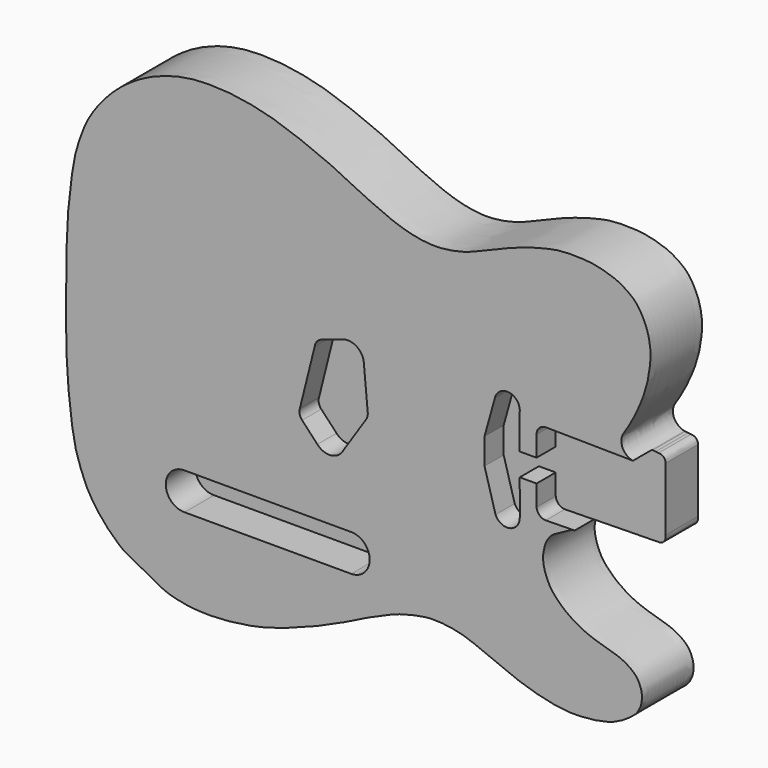
from build123d import *

# Parameters (mm, degrees)
F1_DEPTH = 44.45
F2_DEPTH = 16.51
F3_DEPTH = 25.4


# Not quite as in the source:
# - a feature names something its author has since deleted; it is built from what else it names


with BuildPart() as f1:
    # F0 (on Front) → F1 (new body)
    with BuildSketch(Plane.XZ):
        with BuildLine():
            Line((-36.4628359675, 9.569167666), (-36.4628359675, 27.653967666))
            Line((-36.4628359675, 27.653967666), (-29.3169317005, 53.3077017051))
            ThreePointArc((-29.3169317005, 53.3077017051), (-20.290639837, 59.8672852359), (-12.2146032714, 52.1679531679))
            ThreePointArc((-12.2146032714, 52.1679531679), (-12.1577623785, 51.1793421532), (-12.2134742813, 50.190666873))
            Line((-12.2134742813, 50.190666873), (-12.1998377178, 26.3079138094))
            Line((-12.1998377178, 26.3079138094), (-0.6035441244, 26.3145350559))
            Line((-0.6035441244, 26.3145350559), (-0.6116200717, 40.4585571406))
            ThreePointArc((-0.6116200717, 40.4585571406), (1.2332374634, 44.9781868251), (5.7391212323, 46.856367666))
            Line((5.7391212323, 46.856367666), (65.8569202223, 46.101456937))
            add(Edge.make_bspline(
                [(65.8569202223, 46.101456937), (65.8082198952, 46.111538896), (64.440532792, 46.4005697996), (61.9493146455, 47.2777107227), (58.8086310676, 50.8096057402), (58.0449342483, 53.2991789854), (57.7457666161, 55.8465865019), (58.1162605807, 57.8853867085), (58.8767369784, 60.1253918133), (61.8338810554, 64.2452496747), (64.7748667663, 69.5266396192), (66.9437975867, 73.5325947729), (72.1748619169, 84.4879171866), (75.4157897662, 95.0217528485), (77.0913434636, 102.553719941), (78.8679716791, 117.435063011), (75.0176091289, 132.0874660401), (69.4399127098, 141.1287497127), (66.1646213257, 144.6638685914), (63.8949883169, 146.3744088303), (62.1099414236, 147.7625127314), (59.4477178127, 149.4698385607), (54.8171025343, 152.3289323071), (42.9175321679, 156.1236739531), (32.4036601977, 157.5651964451), (17.2088000215, 157.6253069579), (8.7386710867, 156.0609973015), (-0.497068574, 153.8336518936), (-9.0925484925, 151.2124734508), (-14.4383316219, 149.3290323967), (-22.7118669356, 146.2487000901), (-30.085330014, 142.9097204574), (-39.2612302691, 139.405533864), (-44.8381827502, 136.8638580798), (-51.0647950461, 134.7130453138), (-57.3869608629, 133.2537734899), (-64.5951798295, 132.1353574656), (-72.0653943408, 131.7504818884), (-80.9431789181, 132.7258780715), (-89.4749993511, 134.5505711219), (-99.5171332769, 137.7395440421), (-110.0450246922, 142.4219643584), (-120.9610931472, 147.1972742288), (-134.7691497671, 154.4003080602), (-143.6538012671, 158.4762100092), (-157.5356445432, 164.4053701436), (-175.0197441359, 170.8243226408), (-186.3921154716, 174.3329000019), (-200.859238688, 177.4783450729), (-215.2049744258, 179.3443999642), (-230.3357113691, 179.662308746), (-239.3667204013, 178.8311843075), (-249.7475334686, 176.9580035132), (-258.4388184787, 174.3472655237), (-270.2077546423, 169.617132441), (-281.0330383343, 162.8807350814), (-288.724798983, 156.9716403119), (-296.6119448079, 149.4701577517), (-303.1036787906, 141.6394488957), (-307.9726093768, 134.3784922093), (-311.0811868302, 128.8371006588), (-314.2426482545, 121.1107032616), (-316.6817846786, 114.2377347901), (-319.5777590699, 103.8792354228), (-321.3560431534, 90.7754208806), (-323.3080358572, 75.4582008588), (-324.489070044, 56.0206486034), (-324.9329261688, 30.5273308203), (-325.5213201034, -24.6300824924), (-319.9524725281, -65.9891758085), (-317.0048781693, -76.3928819812), (-311.8939305277, -90.882381175), (-307.2717097261, -98.41395875), (-303.607968046, -103.8373952444), (-299.7301097702, -108.687657352), (-296.0407497518, -113.0005548798), (-290.6753655124, -118.1196416132), (-287.5886005429, -120.701802204), (-285.8139366616, -122.1753017859), (-282.0775126279, -124.3005591876), (-282.0559417692, -124.3111405134)],
                knots=[0.0087884076, 0.0087884076, 0.0087884076, 0.0087884076, 0.0090969709, 0.0174847617, 0.0264572155, 0.033290393, 0.0399451027, 0.0459262298, 0.0522794931, 0.0618231279, 0.0721557838, 0.0812308835, 0.0958978339, 0.1100252966, 0.1217227111, 0.137900103, 0.1545955669, 0.1682230193, 0.1772998584, 0.1842364833, 0.190505402, 0.1977901906, 0.2076124061, 0.2223668275, 0.236629285, 0.2528933764, 0.2654267623, 0.2784218192, 0.2910050259, 0.3011351249, 0.3134791399, 0.3258152578, 0.3389588282, 0.3495071237, 0.360198775, 0.3710109583, 0.382368356, 0.3939634128, 0.4065222933, 0.4190404883, 0.4327282508, 0.4470084074, 0.4618293926, 0.4783570386, 0.49162608, 0.5080146132, 0.5263183465, 0.541010961, 0.5570360296, 0.573418106, 0.5897148303, 0.6025488734, 0.6160172189, 0.6288300734, 0.6438764778, 0.6590024815, 0.672177919, 0.6860518531, 0.6996679541, 0.7120327874, 0.7227283038, 0.7347664787, 0.746248908, 0.759964096, 0.7753743112, 0.79200234, 0.8102768483, 0.8316179392, 0.863706102, 0.8907241456, 0.9045658341, 0.9207868975, 0.9334891204, 0.9441601708, 0.9545570424, 0.9647955615, 0.976344898, 0.984586996, 0.9917273903, 1, 1, 1, 1], degree=3))
            Line((-282.0559417692, -124.3111405134), (-258.0415796527, -137.131692276))
            add(Edge.make_bspline(
                [(-258.0415796527, -137.131692276), (-256.9812734982, -137.60730777), (-254.5368163321, -138.7038040014), (-248.166441932, -140.3729487716), (-242.3794546895, -141.4900264019), (-236.1497706051, -142.2474812095), (-230.1384817638, -142.644410985), (-222.0753688735, -142.5836604529), (-213.2788451825, -142.0513216814), (-204.1233965754, -140.9044073657), (-193.5549385183, -139.0785143182), (-184.0685444079, -136.8051476435), (-170.3880451753, -132.1382147735), (-165.3641554772, -130.3497663035), (-153.6118120984, -125.7592571023), (-147.0728394803, -123.0146200853), (-137.0010009197, -118.4945675196), (-129.0784459928, -114.6510105428), (-121.596863913, -110.6179955538), (-115.7478089519, -108.0091383839), (-107.9588061733, -104.6234424741), (-101.0503452885, -101.4448335986), (-90.4339613221, -97.6341775721), (-79.6953147639, -95.7608277006), (-75.3589076228, -95.0253938848), (-67.4299355422, -94.9965284423), (-60.3742195269, -95.7717114713), (-52.8275417099, -97.3110250627), (-48.1625775991, -98.8063911433), (-43.8435733628, -100.3432338116), (-38.9134501989, -102.5763099343), (-34.6933335006, -104.2081589286), (-30.2312953618, -106.0117013145), (-19.1028962938, -110.7369490595), (-14.4545595602, -112.3932436269), (-9.1997220725, -114.2335320121), (-2.7983386531, -116.2208721773), (4.5026085304, -118.1235376044), (10.8965834624, -119.5511131712), (18.4758168238, -120.6141716364), (24.598947266, -120.9250148011), (29.5677126987, -120.8162411024), (37.1048861789, -120.3821316492), (44.9820022775, -118.892145763), (49.8741103776, -117.7772091505), (55.0626346743, -115.644720613), (60.0089414892, -113.0957899752), (65.1725820337, -109.2090269633), (68.3548395354, -106.6458888457), (70.4895088234, -102.9475783455), (71.5422453481, -100.281139683), (72.0017463543, -97.5568335536), (72.0808342079, -94.0387956371), (71.6944980771, -91.0821214316), (69.7684061365, -86.1635388845), (67.2683067779, -82.9545328161), (63.5028047339, -79.7416668601), (56.4158954866, -75.7597450088), (48.2781096923, -73.8711129189), (34.4644411882, -69.3625330055), (27.0886455851, -65.56386001), (18.580631056, -60.2526006573), (9.9792099458, -51.4002747536), (7.8402919861, -47.2728359169), (5.0003830303, -41.2668597002), (3.7867850092, -34.5772785401), (3.8701411598, -30.6396246836), (5.0033521449, -25.1654101465), (6.3699370481, -21.7160949578), (8.6197695506, -18.510212014), (10.7236537063, -16.5187736502), (14.3347445669, -14.5299828176), (17.9386959277, -12.8416531855), (20.8409763633, -10.9804492983), (23.2458792785, -9.8056742944), (23.4187513062, -9.7102114337), (23.7584072839, -9.6324231495)],
                knots=[0, 0, 0, 0, 0.0104509028, 0.0242148439, 0.0375096501, 0.0508564707, 0.0640936559, 0.0793434464, 0.0953791311, 0.1118285049, 0.1292395879, 0.1466395781, 0.1666689398, 0.1797658562, 0.1983638122, 0.2133183978, 0.2309169625, 0.2472415886, 0.2627173841, 0.2764639729, 0.2919327691, 0.3068931385, 0.3252287313, 0.342846578, 0.3542288202, 0.3690429193, 0.383804903, 0.3986564384, 0.4105476231, 0.4220287423, 0.4345904655, 0.4458034431, 0.4578799613, 0.4765209237, 0.4888143374, 0.5011684739, 0.5152457204, 0.5300254562, 0.543926773, 0.558842121, 0.5721098192, 0.5840292358, 0.5988956147, 0.6142142574, 0.6262966643, 0.6388403029, 0.6517409659, 0.6653651563, 0.6763445695, 0.6872826349, 0.6963714098, 0.705287367, 0.715251395, 0.7246815905, 0.7369009164, 0.7477560737, 0.7596230574, 0.77468036, 0.790653077, 0.8110358725, 0.8266728576, 0.8438531523, 0.8625702891, 0.8742191339, 0.887964822, 0.9019504231, 0.9127616156, 0.925297871, 0.935859507, 0.9462889071, 0.9554699291, 0.9663200571, 0.9771726191, 0.987472648, 0.9957384614, 1, 1, 1, 1], degree=3))
            add(Edge.make_bspline(
                [(23.7584072839, -9.6324231495), (24.3977426434, -9.4750500801), (25.0699117937, -9.3705791469), (25.6709926449, -9.3019980849)],
                knots=[0, 0, 0, 0, 0.4158386089, 0.4158386089, 0.4158386089, 0.4158386089], degree=3))
            Line((25.6709926449, -9.3019980849), (5.7391212323, -9.633232334))
            ThreePointArc((5.7391212323, -9.633232334), (1.3688874104, -7.8765897185), (-0.5864683452, -3.5915785393))
            Line((-0.5864683452, -3.5915785393), (-0.5946112416, 10.6696965847))
            Line((-0.5946112416, 10.6696965847), (-12.190904835, 10.6630753383))
            Line((-12.190904835, 10.6630753383), (-12.1768534091, -13.9462578468))
            ThreePointArc((-12.1768534091, -13.9462578468), (-19.1148449369, -22.4808641066), (-28.8806129965, -17.4207253088))
            Line((-28.8806129965, -17.4207253088), (-36.4628359675, 9.569167666))
        make_face()
        with BuildLine():
            ThreePointArc((-128.7952004173, -60.3126850102), (-115.6391248654, -72.7761053075), (-128.3386472897, -85.7044191818))
            Line((-128.3386472897, -85.7044191818), (-243.2547248342, -85.690169182))
            ThreePointArc((-243.2547248342, -85.690169182), (-256.206382306, -73.1177100909), (-243.50478245, -60.2926751996))
            Line((-243.50478245, -60.2926751996), (-128.7952004173, -60.3126850102))
        make_face(mode=Mode.SUBTRACT)
        with BuildLine():
            ThreePointArc((-134.2817557077, 54.6275939073), (-124.7059028287, 53.5782144041), (-119.6853627977, 45.356758724))
            Line((-119.6853627977, 45.356758724), (-116.971548401, 15.7842517795))
            ThreePointArc((-116.971548401, 15.7842517795), (-116.9677472043, 15.7441490592), (-116.9641860741, 15.7040243085))
            ThreePointArc((-116.9641860741, 15.7040243085), (-117.1459064553, 13.475270746), (-118.047741201, 11.4290403507))
            Line((-118.047741201, 11.4290403507), (-133.7254104602, -12.3960964354))
            ThreePointArc((-133.7254104602, -12.3960964354), (-134.3488126932, -13.4722936549), (-135.0905236842, -14.4706400906))
            ThreePointArc((-135.0905236842, -14.4706400906), (-143.3305428456, -18.3895922885), (-151.669755955, -14.6864008503))
            Line((-151.669755955, -14.6864008503), (-162.2310274393, -3.4697160051))
            ThreePointArc((-162.2310274393, -3.4697160051), (-163.8876183781, -0.3754361904), (-163.7613120315, 3.1321139257))
            Line((-163.7613120315, 3.1321139257), (-153.5126317992, 44.2024849636))
            ThreePointArc((-153.5126317992, 44.2024849636), (-151.9849846776, 47.6611602736), (-148.8337116798, 49.7505666776))
            Line((-148.8337116798, 49.7505666776), (-134.2817557077, 54.6275939073))
        make_face(mode=Mode.SUBTRACT)
        with BuildLine():
            Line((5.7391212323, 46.856367666), (5.7391212323, -9.633232334))
            Line((5.7391212323, -9.633232334), (25.6709926449, -9.3019980849))
            add(Edge.make_bspline(
                [(25.6709926449, -9.3019980849), (25.8183902697, -9.2851805708), (26.6382875045, -9.2012027165), (27.2676087916, -9.1798175126), (28.1531997025, -9.1951219365)],
                knots=[0.4158386089, 0.4158386089, 0.4158386089, 0.4158386089, 0.5178109527, 1, 1, 1, 1], degree=3))
            Line((28.1531997025, -9.1951219365), (70.7962065935, -8.4897931665))
            add(Edge.make_bspline(
                [(70.7962065935, -8.4897931665), (71.232676741, -8.4137848271), (72.0917921847, -8.264175653), (73.2253481248, -7.7493893514), (74.081782899, -6.960448486), (74.5887088859, -6.1968740087), (74.9444226583, -5.4910960126), (75.1332030921, -4.7181760994), (75.1814664562, -3.8039529542), (75.1826551903, -3.0465475377), (75.1832872629, -2.6438205969)],
                knots=[0, 0, 0, 0, 0.1419114588, 0.279327983, 0.411890172, 0.5298881015, 0.6388552662, 0.747869831, 0.8659375686, 1, 1, 1, 1], degree=3))
            Line((75.1832872629, -2.6438205969), (75.1832872629, 40.9117899835))
            add(Edge.make_bspline(
                [(75.1832872629, 40.9117899835), (75.1582605388, 41.2359787721), (75.1048570215, 41.9277521527), (74.7785983937, 43.203857657), (73.7533131604, 44.4131080624), (72.5446714856, 45.144068904), (71.5324744977, 45.3743207151), (70.7226941534, 45.4686528657), (70.298128425, 45.518110967)],
                knots=[0, 0, 0, 0, 0.1496367602, 0.3193038473, 0.5068023143, 0.6825549028, 0.8335643612, 1, 1, 1, 1], degree=3))
            add(Edge.make_bspline(
                [(68.2706800119, 45.7288575578), (68.4233303091, 45.708924893), (69.1640549408, 45.6160309127), (69.7945569841, 45.5615911196), (70.298128425, 45.518110967)],
                knots=[0.4312868789, 0.4312868789, 0.4312868789, 0.4312868789, 0.5457783382, 1, 1, 1, 1], degree=3))
            add(Edge.make_bspline(
                [(68.2706800119, 45.7288575578), (67.6481534532, 45.8016712631), (67.0364111261, 45.8849738266), (66.4454052163, 45.9890671262)],
                knots=[0.0039128198, 0.0039128198, 0.0039128198, 0.0039128198, 0.007561972, 0.007561972, 0.007561972, 0.007561972], degree=3))
            add(Edge.make_bspline(
                [(66.4454052163, 45.9890671262), (66.2467753316, 46.0240516158), (66.0504877293, 46.0613845233), (65.8569202223, 46.101456937)],
                knots=[0.007561972, 0.007561972, 0.007561972, 0.007561972, 0.0087884076, 0.0087884076, 0.0087884076, 0.0087884076], degree=3))
            Line((65.8569202223, 46.101456937), (5.7391212323, 46.856367666))
        make_face()
        with BuildLine():
            Line((-243.2547248342, -85.690169182), (-128.3386472897, -85.7044191818))
            ThreePointArc((-128.3386472897, -85.7044191818), (-115.6391248654, -72.7761053075), (-128.7952004173, -60.3126850102))
            Line((-128.7952004173, -60.3126850102), (-243.50478245, -60.2926751996))
            ThreePointArc((-243.50478245, -60.2926751996), (-256.206382306, -73.1177100909), (-243.2547248342, -85.690169182))
        make_face()
        with BuildLine():
            Line((-116.971548401, 15.7842517795), (-119.6853627977, 45.356758724))
            ThreePointArc((-119.6853627977, 45.356758724), (-124.7059028287, 53.5782144041), (-134.2817557077, 54.6275939073))
            Line((-134.2817557077, 54.6275939073), (-148.8337116798, 49.7505666776))
            ThreePointArc((-148.8337116798, 49.7505666776), (-151.9849846776, 47.6611602736), (-153.5126317992, 44.2024849636))
            Line((-153.5126317992, 44.2024849636), (-163.7613120315, 3.1321139257))
            ThreePointArc((-163.7613120315, 3.1321139257), (-163.8876183781, -0.3754361904), (-162.2310274393, -3.4697160051))
            Line((-162.2310274393, -3.4697160051), (-151.669755955, -14.6864008503))
            ThreePointArc((-151.669755955, -14.6864008503), (-143.3305428456, -18.3895922885), (-135.0905236842, -14.4706400906))
            Line((-135.0905236842, -14.4706400906), (-133.7254104602, -12.3960964354))
            Line((-133.7254104602, -12.3960964354), (-118.047741201, 11.4290403507))
            ThreePointArc((-118.047741201, 11.4290403507), (-117.1459064553, 13.475270746), (-116.9641860741, 15.7040243085))
            ThreePointArc((-116.9641860741, 15.7040243085), (-116.9677472043, 15.7441490592), (-116.971548401, 15.7842517795))
        make_face()
        with BuildLine():
            Line((-29.3169317005, 53.3077017051), (-36.4628359675, 27.653967666))
            Line((-36.4628359675, 27.653967666), (-36.4628359675, 9.569167666))
            Line((-36.4628359675, 9.569167666), (-28.8806129965, -17.4207253088))
            ThreePointArc((-28.8806129965, -17.4207253088), (-19.1148449369, -22.4808641066), (-12.1768534091, -13.9462578468))
            Line((-12.1768534091, -13.9462578468), (-12.190904835, 10.6630753383))
            Line((-12.190904835, 10.6630753383), (-12.1998377178, 26.3079138094))
            Line((-12.1998377178, 26.3079138094), (-12.2134742813, 50.190666873))
            Line((-12.2134742813, 50.190666873), (-12.2146032714, 52.1679531679))
            ThreePointArc((-12.2146032714, 52.1679531679), (-20.290639837, 59.8672852359), (-29.3169317005, 53.3077017051))
        make_face()
        with BuildLine():
            Line((-12.1998377178, 26.3079138094), (-12.190904835, 10.6630753383))
            Line((-12.190904835, 10.6630753383), (-0.5946112416, 10.6696965847))
            Line((-0.5946112416, 10.6696965847), (-0.5864683452, -3.5915785393))
            ThreePointArc((-0.5864683452, -3.5915785393), (1.3688874104, -7.8765897185), (5.7391212323, -9.633232334))
            Line((5.7391212323, -9.633232334), (5.7391212323, 46.856367666))
            ThreePointArc((5.7391212323, 46.856367666), (1.2332374634, 44.9781868251), (-0.6116200717, 40.4585571406))
            Line((-0.6116200717, 40.4585571406), (-0.6035441244, 26.3145350559))
            Line((-0.6035441244, 26.3145350559), (-12.1998377178, 26.3079138094))
        make_face()
        with BuildLine():
            add(Edge.make_bspline(
                [(66.4454052163, 45.9890671262), (67.0705274115, 45.896505303), (67.6956496067, 45.8039434797), (68.2706800119, 45.7288575578)],
                knots=[0, 0, 0, 0, 0.4312868789, 0.4312868789, 0.4312868789, 0.4312868789], degree=3))
            add(Edge.make_bspline(
                [(68.2706800119, 45.7288575578), (67.6481534532, 45.8016712631), (67.0364111261, 45.8849738266), (66.4454052163, 45.9890671262)],
                knots=[0.0039128198, 0.0039128198, 0.0039128198, 0.0039128198, 0.007561972, 0.007561972, 0.007561972, 0.007561972], degree=3))
        make_face()
    extrude(amount=-F1_DEPTH)

    # F0 (on Front) → F2 (cut)
    with BuildSketch(Plane.XZ):
        with BuildLine():
            Line((-116.971548401, 15.7842517795), (-119.6853627977, 45.356758724))
            ThreePointArc((-119.6853627977, 45.356758724), (-124.7059028287, 53.5782144041), (-134.2817557077, 54.6275939073))
            Line((-134.2817557077, 54.6275939073), (-148.8337116798, 49.7505666776))
            ThreePointArc((-148.8337116798, 49.7505666776), (-151.9849846776, 47.6611602736), (-153.5126317992, 44.2024849636))
            Line((-153.5126317992, 44.2024849636), (-163.7613120315, 3.1321139257))
            ThreePointArc((-163.7613120315, 3.1321139257), (-163.8876183781, -0.3754361904), (-162.2310274393, -3.4697160051))
            Line((-162.2310274393, -3.4697160051), (-151.669755955, -14.6864008503))
            ThreePointArc((-151.669755955, -14.6864008503), (-143.3305428456, -18.3895922885), (-135.0905236842, -14.4706400906))
            Line((-135.0905236842, -14.4706400906), (-133.7254104602, -12.3960964354))
            Line((-133.7254104602, -12.3960964354), (-118.047741201, 11.4290403507))
            ThreePointArc((-118.047741201, 11.4290403507), (-117.1459064553, 13.475270746), (-116.9641860741, 15.7040243085))
            ThreePointArc((-116.9641860741, 15.7040243085), (-116.9677472043, 15.7441490592), (-116.971548401, 15.7842517795))
        make_face()
        with BuildLine():
            Line((-29.3169317005, 53.3077017051), (-36.4628359675, 27.653967666))
            Line((-36.4628359675, 27.653967666), (-36.4628359675, 9.569167666))
            Line((-36.4628359675, 9.569167666), (-28.8806129965, -17.4207253088))
            ThreePointArc((-28.8806129965, -17.4207253088), (-19.1148449369, -22.4808641066), (-12.1768534091, -13.9462578468))
            Line((-12.1768534091, -13.9462578468), (-12.190904835, 10.6630753383))
            Line((-12.190904835, 10.6630753383), (-12.1998377178, 26.3079138094))
            Line((-12.1998377178, 26.3079138094), (-12.2134742813, 50.190666873))
            Line((-12.2134742813, 50.190666873), (-12.2146032714, 52.1679531679))
            ThreePointArc((-12.2146032714, 52.1679531679), (-20.290639837, 59.8672852359), (-29.3169317005, 53.3077017051))
        make_face()
        with BuildLine():
            Line((-12.1998377178, 26.3079138094), (-12.190904835, 10.6630753383))
            Line((-12.190904835, 10.6630753383), (-0.5946112416, 10.6696965847))
            Line((-0.5946112416, 10.6696965847), (-0.5864683452, -3.5915785393))
            ThreePointArc((-0.5864683452, -3.5915785393), (1.3688874104, -7.8765897185), (5.7391212323, -9.633232334))
            Line((5.7391212323, -9.633232334), (5.7391212323, 46.856367666))
            ThreePointArc((5.7391212323, 46.856367666), (1.2332374634, 44.9781868251), (-0.6116200717, 40.4585571406))
            Line((-0.6116200717, 40.4585571406), (-0.6035441244, 26.3145350559))
            Line((-0.6035441244, 26.3145350559), (-12.1998377178, 26.3079138094))
        make_face()
        with BuildLine():
            Line((5.7391212323, 46.856367666), (5.7391212323, -9.633232334))
            Line((5.7391212323, -9.633232334), (25.6709926449, -9.3019980849))
            add(Edge.make_bspline(
                [(25.6709926449, -9.3019980849), (25.8183902697, -9.2851805708), (26.6382875045, -9.2012027165), (27.2676087916, -9.1798175126), (28.1531997025, -9.1951219365)],
                knots=[0.4158386089, 0.4158386089, 0.4158386089, 0.4158386089, 0.5178109527, 1, 1, 1, 1], degree=3))
            Line((28.1531997025, -9.1951219365), (70.7962065935, -8.4897931665))
            add(Edge.make_bspline(
                [(70.7962065935, -8.4897931665), (71.232676741, -8.4137848271), (72.0917921847, -8.264175653), (73.2253481248, -7.7493893514), (74.081782899, -6.960448486), (74.5887088859, -6.1968740087), (74.9444226583, -5.4910960126), (75.1332030921, -4.7181760994), (75.1814664562, -3.8039529542), (75.1826551903, -3.0465475377), (75.1832872629, -2.6438205969)],
                knots=[0, 0, 0, 0, 0.1419114588, 0.279327983, 0.411890172, 0.5298881015, 0.6388552662, 0.747869831, 0.8659375686, 1, 1, 1, 1], degree=3))
            Line((75.1832872629, -2.6438205969), (75.1832872629, 40.9117899835))
            add(Edge.make_bspline(
                [(75.1832872629, 40.9117899835), (75.1582605388, 41.2359787721), (75.1048570215, 41.9277521527), (74.7785983937, 43.203857657), (73.7533131604, 44.4131080624), (72.5446714856, 45.144068904), (71.5324744977, 45.3743207151), (70.7226941534, 45.4686528657), (70.298128425, 45.518110967)],
                knots=[0, 0, 0, 0, 0.1496367602, 0.3193038473, 0.5068023143, 0.6825549028, 0.8335643612, 1, 1, 1, 1], degree=3))
            add(Edge.make_bspline(
                [(68.2706800119, 45.7288575578), (68.4233303091, 45.708924893), (69.1640549408, 45.6160309127), (69.7945569841, 45.5615911196), (70.298128425, 45.518110967)],
                knots=[0.4312868789, 0.4312868789, 0.4312868789, 0.4312868789, 0.5457783382, 1, 1, 1, 1], degree=3))
            add(Edge.make_bspline(
                [(68.2706800119, 45.7288575578), (67.6481534532, 45.8016712631), (67.0364111261, 45.8849738266), (66.4454052163, 45.9890671262)],
                knots=[0.0039128198, 0.0039128198, 0.0039128198, 0.0039128198, 0.007561972, 0.007561972, 0.007561972, 0.007561972], degree=3))
            add(Edge.make_bspline(
                [(66.4454052163, 45.9890671262), (66.2467753316, 46.0240516158), (66.0504877293, 46.0613845233), (65.8569202223, 46.101456937)],
                knots=[0.007561972, 0.007561972, 0.007561972, 0.007561972, 0.0087884076, 0.0087884076, 0.0087884076, 0.0087884076], degree=3))
            Line((65.8569202223, 46.101456937), (5.7391212323, 46.856367666))
        make_face()
        with BuildLine():
            add(Edge.make_bspline(
                [(66.4454052163, 45.9890671262), (67.0705274115, 45.896505303), (67.6956496067, 45.8039434797), (68.2706800119, 45.7288575578)],
                knots=[0, 0, 0, 0, 0.4312868789, 0.4312868789, 0.4312868789, 0.4312868789], degree=3))
            add(Edge.make_bspline(
                [(68.2706800119, 45.7288575578), (67.6481534532, 45.8016712631), (67.0364111261, 45.8849738266), (66.4454052163, 45.9890671262)],
                knots=[0.0039128198, 0.0039128198, 0.0039128198, 0.0039128198, 0.007561972, 0.007561972, 0.007561972, 0.007561972], degree=3))
        make_face()
    extrude(amount=-F2_DEPTH, mode=Mode.SUBTRACT)

    # F0 (on Front) → F3 (cut)
    with BuildSketch(Plane.XZ):
        with BuildLine():
            Line((-243.2547248342, -85.690169182), (-128.3386472897, -85.7044191818))
            ThreePointArc((-128.3386472897, -85.7044191818), (-115.6391248654, -72.7761053075), (-128.7952004173, -60.3126850102))
            Line((-128.7952004173, -60.3126850102), (-243.50478245, -60.2926751996))
            ThreePointArc((-243.50478245, -60.2926751996), (-256.206382306, -73.1177100909), (-243.2547248342, -85.690169182))
        make_face()
    extrude(amount=-F3_DEPTH, mode=Mode.SUBTRACT)


solid = f1.part
